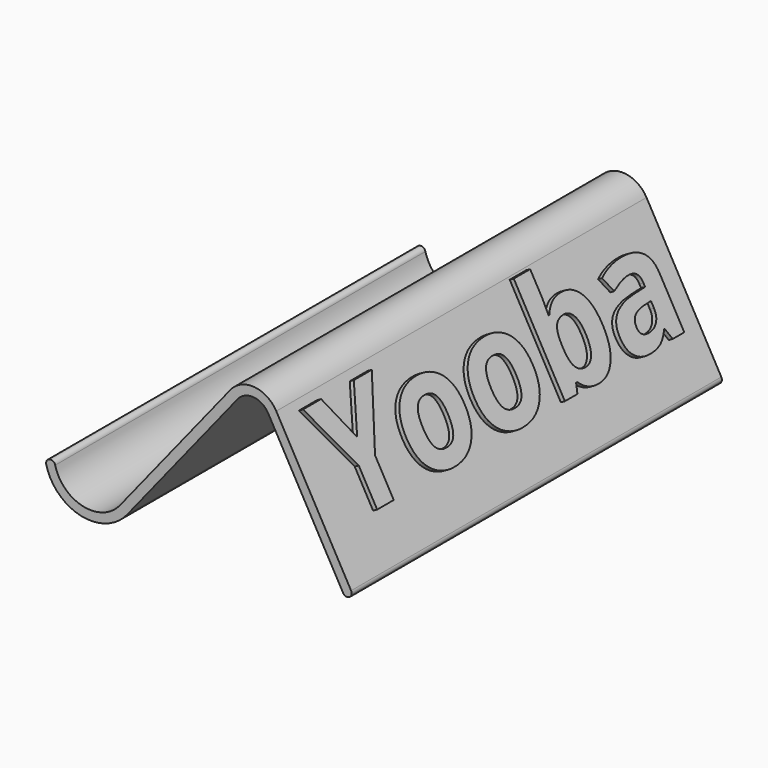
from build123d import *

# Parameters (mm, degrees)
F1_DEPTH     = 100
F2_TEXT_SIZE = 29.7612896559
F3_DEPTH     = 1


# Not quite as in the source:
# - Text() gives the source's letters only with a copy of the font that has no kerning and outlines rounded to 1/6400 em; it was checked with that copy


with BuildPart() as f1:
    # F0 (on Front) → F1 (new body)
    with BuildSketch(Plane.XZ):
        with BuildLine():
            Line((-5.5691709353, 29.7125615033), (-29.4255502831, 0))
            ThreePointArc((-29.4255502831, 0), (-37.3779461859, -2.8055614979), (-43.4255502831, 3.0713646201))
            ThreePointArc((-43.4255502831, 3.0713646201), (-44.6379428305, 3.7994472467), (-45.366025457, 2.5870546993))
            ThreePointArc((-45.366025457, 2.5870546993), (-37.8065203355, -4.7591029483), (-27.866025457, -1.2521510759))
            Line((-27.866025457, -1.2521510759), (-4.0096461092, 28.4604104274))
            ThreePointArc((-4.0096461092, 28.4604104274), (-0.5585863113, 29.9423056194), (2.5997686299, 27.9099126568))
            Line((2.5997686299, 27.9099126568), (18.7697634585, -0.9769021906))
            ThreePointArc((18.7697634585, -0.9769021906), (20.1308058255, -1.361042367), (20.5149460019, 0))
            Line((20.5149460019, 0), (4.3449511734, 28.8868148474))
            ThreePointArc((4.3449511734, 28.8868148474), (-0.3925812384, 31.9354042913), (-5.5691709353, 29.7125615033))
        make_face()
    extrude(amount=F1_DEPTH)

    # F2 (on face) → F3 (join)
    with BuildSketch(Plane(origin=(15.620398432, 0, 8.743842587), x_dir=(0, 1, 0), z_dir=(0.8725912717, 0, 0.4884510953))):
        with Locations((-95, -0.0205478443)):
            Text('Yooba', F2_TEXT_SIZE, font='Open Sans', font_style=FontStyle.BOLD, text_align=(TextAlign.LEFT, TextAlign.BOTTOM))
    extrude(amount=F3_DEPTH)


solid = f1.part
